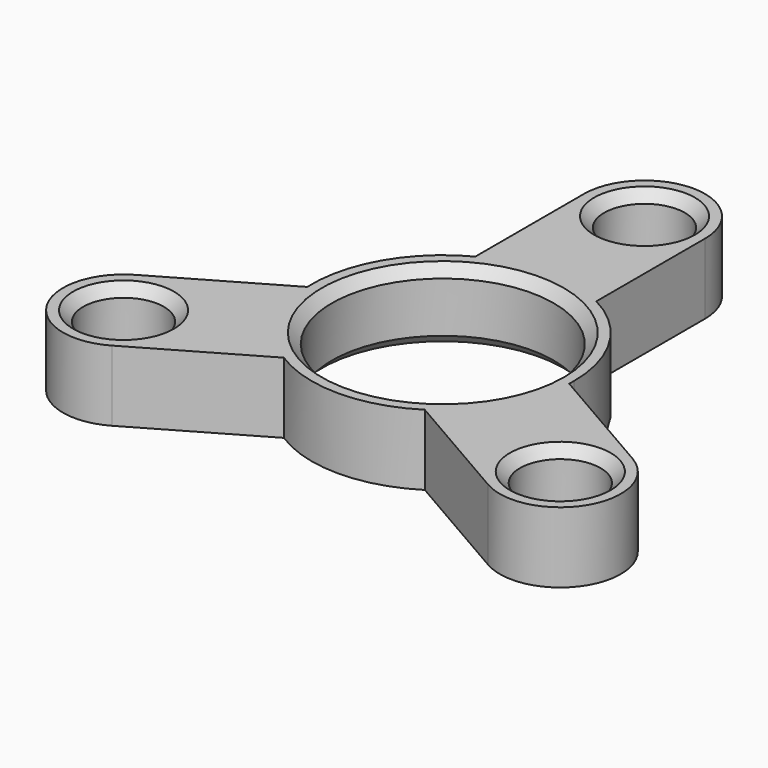
from build123d import *

# Parameters (mm, degrees)
F0_R     = 11
F0_R_2   = 4
F1_DEPTH = 3.5
F2_SIZE  = 1


# Not quite as in the source:
# - a feature names something its author has since deleted; it is built from what else it names


with BuildPart() as f1:
    # F0 (on Top) → F1 (new body, symmetric)
    with BuildSketch(Plane.XY):
        with BuildLine():
            ThreePointArc((-6, 11.5325625947), (0, 13), (6, 11.5325625947))
            Line((6, 11.5325625947), (6, 25))
            ThreePointArc((6, 25), (0, 19), (-6, 25))
            Line((-6, 25), (-6, 11.5325625947))
        make_face()
        with BuildLine():
            ThreePointArc((-6.9874921777, -10.96243372), (-11.2583302492, -6.5), (-12.9874921777, -0.5701288746))
            Line((-12.9874921777, -0.5701288746), (-24.6506350946, -7.3038475773))
            ThreePointArc((-24.6506350946, -7.3038475773), (-18.6506350946, -7.3038475773), (-15.6506350946, -12.5))
            ThreePointArc((-15.6506350946, -12.5), (-16.4544826719, -15.5), (-18.6506350946, -17.6961524227))
            Line((-18.6506350946, -17.6961524227), (-6.9874921777, -10.96243372))
        make_face()
        with BuildLine():
            Line((24.6506350946, -7.3038475773), (12.9874921777, -0.5701288746))
            ThreePointArc((12.9874921777, -0.5701288746), (11.2583302492, -6.5), (6.9874921777, -10.96243372))
            Line((6.9874921777, -10.96243372), (18.6506350946, -17.6961524227))
            ThreePointArc((18.6506350946, -17.6961524227), (16.4544826719, -9.5), (24.6506350946, -7.3038475773))
        make_face()
        with BuildLine():
            ThreePointArc((12.9874921777, -0.5701288746), (12.9968726683, -0.2851330301), (13, 0))
            ThreePointArc((13, 0), (11.1130553854, 6.7453687816), (6, 11.5325625947))
            ThreePointArc((6, 11.5325625947), (0, 13), (-6, 11.5325625947))
            ThreePointArc((-6, 11.5325625947), (-11.2583302492, 6.5), (-12.9874921777, -0.5701288746))
            ThreePointArc((-12.9874921777, -0.5701288746), (-11.2583302492, -6.5), (-6.9874921777, -10.96243372))
            ThreePointArc((-6.9874921777, -10.96243372), (0, -13), (6.9874921777, -10.96243372))
            ThreePointArc((6.9874921777, -10.96243372), (11.2583302492, -6.5), (12.9874921777, -0.5701288746))
        make_face()
        Circle(F0_R, mode=Mode.SUBTRACT)
        with BuildLine():
            ThreePointArc((-6, 25), (0, 19), (6, 25))
            ThreePointArc((6, 25), (0, 31), (-6, 25))
        make_face()
        with Locations((0, 25)):
            Circle(F0_R_2, mode=Mode.SUBTRACT)
        with BuildLine():
            ThreePointArc((-15.6506350946, -12.5), (-18.6506350946, -7.3038475773), (-24.6506350946, -7.3038475773))
            ThreePointArc((-24.6506350946, -7.3038475773), (-26.8467875173, -15.5), (-18.6506350946, -17.6961524227))
            ThreePointArc((-18.6506350946, -17.6961524227), (-16.4544826719, -15.5), (-15.6506350946, -12.5))
        make_face()
        with Locations((-21.6506350946, -12.5)):
            Circle(F0_R_2, mode=Mode.SUBTRACT)
        with BuildLine():
            ThreePointArc((27.6506350946, -12.5), (26.8467875173, -9.5), (24.6506350946, -7.3038475773))
            ThreePointArc((24.6506350946, -7.3038475773), (16.4544826719, -9.5), (18.6506350946, -17.6961524227))
            ThreePointArc((18.6506350946, -17.6961524227), (24.6506350946, -17.6961524227), (27.6506350946, -12.5))
        make_face()
        with Locations((21.6506350946, -12.5)):
            Circle(F0_R_2, mode=Mode.SUBTRACT)
    extrude(amount=F1_DEPTH, both=True)

    # F2
    f2_edges = [f1.edges().sort_by_distance(p)[0] for p in [
        (-4, 25, 3.5),
        (-11, 0, 3.5),
        (-25.650635, -12.5, 3.5),
        (17.650635, -12.5, 3.5),
        (-25.650635, -12.5, -3.5),
        (-11, 0, -3.5),
        (17.650635, -12.5, -3.5),
        (-4, 25, -3.5),
    ]]
    chamfer(f2_edges, length=F2_SIZE)


solid = f1.part
